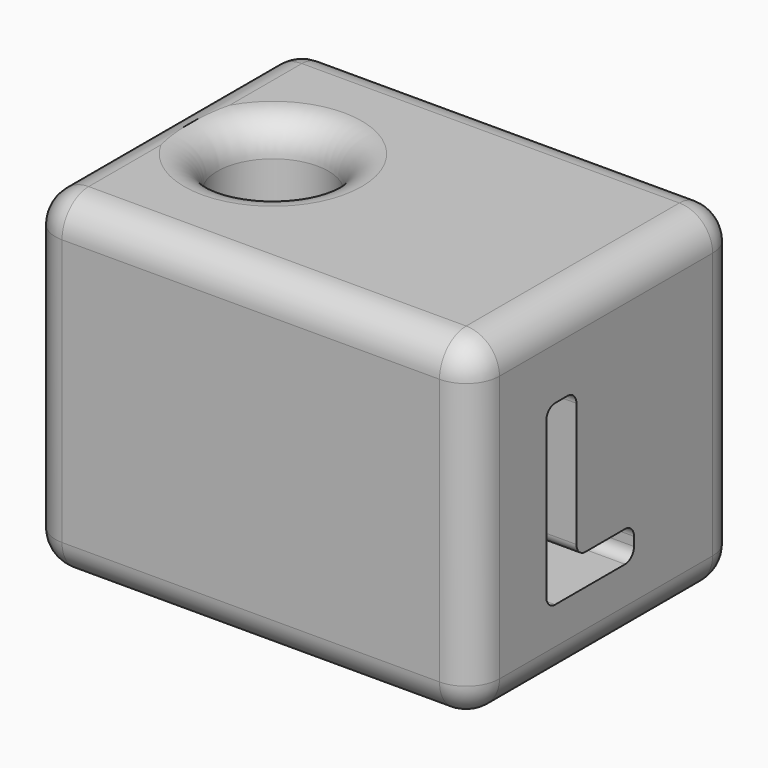
from build123d import *

# Parameters (mm, degrees)
F0_W         = 50.8
F0_H         = 38.1
F1_DEPTH     = 38.1
F2_R         = 6.35
F3_DEPTH     = 38.101
F4_T1_DEPTH  = 43.18
F4_T3_DEPTH  = 30.48
F4_T5_DEPTH  = 30.48
F4_S9_W      = 3.81
F4_S9_H      = 3.81
F4_T10_DEPTH = 3.81
F4_S15_W     = 3.81
F4_S15_H     = 3.81
F4_T16_DEPTH = 3.81
F4_S21_W     = 3.81
F4_S21_H     = 3.81
F4_T22_DEPTH = 3.81
F4_S27_W     = 3.81
F4_S27_H     = 3.81
F4_T28_DEPTH = 3.81
F4_S33_W     = 3.81
F4_S33_H     = 3.81
F4_T34_DEPTH = 3.81
F4_S39_W     = 3.81
F4_S39_H     = 3.81
F4_T40_DEPTH = 3.81
F4_S45_W     = 3.81
F4_S45_H     = 3.81
F4_T46_DEPTH = 3.81
F4_S51_W     = 3.81
F4_S51_H     = 3.81
F4_T52_DEPTH = 3.81
F5_TEXT_SIZE = 28.4437594625
F6_DEPTH     = 50.8010001
F7_R         = 1.27
F8_TEXT_SIZE = 26.0072152337
F9_DEPTH     = 1.27


# Not quite as in the source:
# - a fillet or chamfer that OpenCascade refuses, or shapes differently, is made with other operations: its cross-section is extruded or revolved along the edge and cut away or added
# - Text() gives the source's letters only with a copy of the font that has no kerning and outlines rounded to 1/6400 em; it was checked with that copy


with BuildPart() as f1:
    # F0 (on Top) → F1 (new body)
    with BuildSketch(Plane.XY):
        with Locations((25.4, 19.05)):
            Rectangle(F0_W, F0_H)
    extrude(amount=F1_DEPTH)

    # F2 (on face) → F3 (cut, through all)
    with BuildSketch(Plane.XY.offset(38.1)):
        with Locations((12.7, 19.05)):
            Circle(F2_R)
    extrude(amount=-F3_DEPTH, mode=Mode.SUBTRACT)

    # F4: fillet of radius 3.81 on 14 edges, made by hand

    # F4_s2 → F4_t1 (cut)
    with BuildSketch(Plane.YZ.offset(3.81)):
        with BuildLine():
            ThreePointArc((0, 34.29), (1.1159231637, 36.9840768363), (3.81, 38.1))
            Line((3.81, 38.1), (0, 38.1))
            Line((0, 38.1), (0, 34.29))
        make_face()
        with BuildLine():
            ThreePointArc((38.1, 34.29), (36.9840768363, 36.9840768363), (34.29, 38.1))
            Line((34.29, 38.1), (38.1, 38.1))
            Line((38.1, 38.1), (38.1, 34.29))
        make_face()
        with BuildLine():
            ThreePointArc((38.1, 3.81), (36.9840768363, 1.1159231637), (34.29, 0))
            Line((34.29, 0), (38.1, 0))
            Line((38.1, 0), (38.1, 3.81))
        make_face()
        with BuildLine():
            ThreePointArc((0, 3.81), (1.1159231637, 1.1159231637), (3.81, 0))
            Line((3.81, 0), (0, 0))
            Line((0, 0), (0, 3.81))
        make_face()
    extrude(amount=F4_T1_DEPTH, mode=Mode.SUBTRACT)

    # F4_s4 → F4_t3 (cut)
    with BuildSketch(Plane.XZ.offset(-34.29)):
        with BuildLine():
            ThreePointArc((0, 34.29), (1.1159231637, 36.9840768363), (3.81, 38.1))
            Line((3.81, 38.1), (0, 38.1))
            Line((0, 38.1), (0, 34.29))
        make_face()
        with BuildLine():
            ThreePointArc((46.99, 38.1), (49.6840768363, 36.9840768363), (50.8, 34.29))
            Line((50.8, 34.29), (50.8, 38.1))
            Line((50.8, 38.1), (46.99, 38.1))
        make_face()
        with BuildLine():
            ThreePointArc((0, 3.81), (1.1159231637, 1.1159231637), (3.81, 0))
            Line((3.81, 0), (0, 0))
            Line((0, 0), (0, 3.81))
        make_face()
        with BuildLine():
            ThreePointArc((46.99, 0), (49.6840768363, 1.1159231637), (50.8, 3.81))
            Line((50.8, 3.81), (50.8, 0))
            Line((50.8, 0), (46.99, 0))
        make_face()
    extrude(amount=F4_T3_DEPTH, mode=Mode.SUBTRACT)

    # F4_s6 → F4_t5 (cut)
    with BuildSketch(Plane.XY.offset(3.81)):
        with BuildLine():
            ThreePointArc((46.99, 0), (49.6840768363, 1.1159231637), (50.8, 3.81))
            Line((50.8, 3.81), (50.8, 0))
            Line((50.8, 0), (46.99, 0))
        make_face()
        with BuildLine():
            ThreePointArc((46.99, 38.1), (49.6840768363, 36.9840768363), (50.8, 34.29))
            Line((50.8, 34.29), (50.8, 38.1))
            Line((50.8, 38.1), (46.99, 38.1))
        make_face()
        with BuildLine():
            ThreePointArc((0, 34.29), (1.1159231637, 36.9840768363), (3.81, 38.1))
            Line((3.81, 38.1), (0, 38.1))
            Line((0, 38.1), (0, 34.29))
        make_face()
        with BuildLine():
            ThreePointArc((0, 3.81), (1.1159231637, 1.1159231637), (3.81, 0))
            Line((3.81, 0), (0, 0))
            Line((0, 0), (0, 3.81))
        make_face()
    extrude(amount=F4_T5_DEPTH, mode=Mode.SUBTRACT)


with BuildPart() as f4_tool8:
    # F4_s9 → F4_t10 (new body)
    with BuildSketch(Plane.YZ.offset(3.81)):
        with Locations((1.905, 36.195)):
            Rectangle(F4_S9_W, F4_S9_H)
    extrude(amount=-F4_T10_DEPTH)

    # F4_s11 → F4_t12 (revolve, cut)
    with BuildSketch(Plane(origin=(3.81, 3.81, 34.29), x_dir=(0, 0.7071067812, -0.7071067812), z_dir=(0, 0.7071067812, 0.7071067812))):
        with BuildLine():
            ThreePointArc((0, -3.81), (3.81, 0), (0, 3.81))
            Line((0, 3.81), (0, -3.81))
        make_face()
    revolve(axis=Axis((3.81, 3.81, 34.29), (-1, 0, 0)), mode=Mode.SUBTRACT)


with BuildPart() as f1_1:
    add(f1.part)

    # F4_t7: cut F4_tool8
    add(f4_tool8.part, mode=Mode.SUBTRACT)


with BuildPart() as f4_tool14:
    # F4_s15 → F4_t16 (new body)
    with BuildSketch(Plane.XZ.offset(-3.81)):
        with Locations((48.895, 36.195)):
            Rectangle(F4_S15_W, F4_S15_H)
    extrude(amount=F4_T16_DEPTH)

    # F4_s17 → F4_t18 (revolve, cut)
    with BuildSketch(Plane(origin=(46.99, 3.81, 34.29), x_dir=(-0.7071067812, 0, -0.7071067812), z_dir=(-0.7071067812, 0, 0.7071067812))):
        with BuildLine():
            ThreePointArc((0, -3.81), (3.81, 0), (0, 3.81))
            Line((0, 3.81), (0, -3.81))
        make_face()
    revolve(axis=Axis((46.99, 3.81, 34.29), (0, -1, 0)), mode=Mode.SUBTRACT)


with BuildPart() as f1_2:
    add(f1_1.part)

    # F4_t13: cut F4_tool14
    add(f4_tool14.part, mode=Mode.SUBTRACT)


with BuildPart() as f4_tool20:
    # F4_s21 → F4_t22 (new body)
    with BuildSketch(Plane.YZ.offset(3.81)):
        with Locations((36.195, 36.195)):
            Rectangle(F4_S21_W, F4_S21_H)
    extrude(amount=-F4_T22_DEPTH)

    # F4_s23 → F4_t24 (revolve, cut)
    with BuildSketch(Plane(origin=(3.81, 34.29, 34.29), x_dir=(0, -0.7071067812, -0.7071067812), z_dir=(0, 0.7071067812, -0.7071067812))):
        with BuildLine():
            ThreePointArc((0, -3.81), (3.81, 0), (0, 3.81))
            Line((0, 3.81), (0, -3.81))
        make_face()
    revolve(axis=Axis((3.81, 34.29, 34.29), (-1, 0, 0)), mode=Mode.SUBTRACT)


with BuildPart() as f1_3:
    add(f1_2.part)

    # F4_t19: cut F4_tool20
    add(f4_tool20.part, mode=Mode.SUBTRACT)


with BuildPart() as f4_tool26:
    # F4_s27 → F4_t28 (new body)
    with BuildSketch(Plane.XZ.offset(-34.29)):
        with Locations((48.895, 36.195)):
            Rectangle(F4_S27_W, F4_S27_H)
    extrude(amount=-F4_T28_DEPTH)

    # F4_s29 → F4_t30 (revolve, cut)
    with BuildSketch(Plane(origin=(46.99, 34.29, 34.29), x_dir=(-0.7071067812, 0, -0.7071067812), z_dir=(0.7071067812, 0, -0.7071067812))):
        with BuildLine():
            ThreePointArc((0, -3.81), (3.81, 0), (0, 3.81))
            Line((0, 3.81), (0, -3.81))
        make_face()
    revolve(axis=Axis((46.99, 34.29, 34.29), (0, 1, 0)), mode=Mode.SUBTRACT)


with BuildPart() as f1_4:
    add(f1_3.part)

    # F4_t25: cut F4_tool26
    add(f4_tool26.part, mode=Mode.SUBTRACT)


with BuildPart() as f4_tool32:
    # F4_s33 → F4_t34 (new body)
    with BuildSketch(Plane.XZ.offset(-34.29)):
        with Locations((48.895, 1.905)):
            Rectangle(F4_S33_W, F4_S33_H)
    extrude(amount=-F4_T34_DEPTH)

    # F4_s35 → F4_t36 (revolve, cut)
    with BuildSketch(Plane(origin=(46.99, 34.29, 3.81), x_dir=(-0.7071067812, 0, 0.7071067812), z_dir=(-0.7071067812, 0, -0.7071067812))):
        with BuildLine():
            ThreePointArc((0, -3.81), (3.81, 0), (0, 3.81))
            Line((0, 3.81), (0, -3.81))
        make_face()
    revolve(axis=Axis((46.99, 34.29, 3.81), (0, 1, 0)), mode=Mode.SUBTRACT)


with BuildPart() as f1_5:
    add(f1_4.part)

    # F4_t31: cut F4_tool32
    add(f4_tool32.part, mode=Mode.SUBTRACT)


with BuildPart() as f4_tool38:
    # F4_s39 → F4_t40 (new body)
    with BuildSketch(Plane.YZ.offset(3.81)):
        with Locations((36.195, 1.905)):
            Rectangle(F4_S39_W, F4_S39_H)
    extrude(amount=-F4_T40_DEPTH)

    # F4_s41 → F4_t42 (revolve, cut)
    with BuildSketch(Plane(origin=(3.81, 34.29, 3.81), x_dir=(0, -0.7071067812, 0.7071067812), z_dir=(0, -0.7071067812, -0.7071067812))):
        with BuildLine():
            ThreePointArc((0, -3.81), (3.81, 0), (0, 3.81))
            Line((0, 3.81), (0, -3.81))
        make_face()
    revolve(axis=Axis((3.81, 34.29, 3.81), (-1, 0, 0)), mode=Mode.SUBTRACT)


with BuildPart() as f1_6:
    add(f1_5.part)

    # F4_t37: cut F4_tool38
    add(f4_tool38.part, mode=Mode.SUBTRACT)


with BuildPart() as f4_tool44:
    # F4_s45 → F4_t46 (new body)
    with BuildSketch(Plane.YZ.offset(3.81)):
        with Locations((1.905, 1.905)):
            Rectangle(F4_S45_W, F4_S45_H)
    extrude(amount=-F4_T46_DEPTH)

    # F4_s47 → F4_t48 (revolve, cut)
    with BuildSketch(Plane(origin=(3.81, 3.81, 3.81), x_dir=(0, 0.7071067812, 0.7071067812), z_dir=(0, -0.7071067812, 0.7071067812))):
        with BuildLine():
            ThreePointArc((0, -3.81), (3.81, 0), (0, 3.81))
            Line((0, 3.81), (0, -3.81))
        make_face()
    revolve(axis=Axis((3.81, 3.81, 3.81), (-1, 0, 0)), mode=Mode.SUBTRACT)


with BuildPart() as f1_7:
    add(f1_6.part)

    # F4_t43: cut F4_tool44
    add(f4_tool44.part, mode=Mode.SUBTRACT)


with BuildPart() as f4_tool50:
    # F4_s51 → F4_t52 (new body)
    with BuildSketch(Plane.XZ.offset(-3.81)):
        with Locations((48.895, 1.905)):
            Rectangle(F4_S51_W, F4_S51_H)
    extrude(amount=F4_T52_DEPTH)

    # F4_s53 → F4_t54 (revolve, cut)
    with BuildSketch(Plane(origin=(46.99, 3.81, 3.81), x_dir=(-0.7071067812, 0, 0.7071067812), z_dir=(0.7071067812, 0, 0.7071067812))):
        with BuildLine():
            ThreePointArc((0, -3.81), (3.81, 0), (0, 3.81))
            Line((0, 3.81), (0, -3.81))
        make_face()
    revolve(axis=Axis((46.99, 3.81, 3.81), (0, -1, 0)), mode=Mode.SUBTRACT)


with BuildPart() as f1_8:
    add(f1_7.part)

    # F4_t49: cut F4_tool50
    add(f4_tool50.part, mode=Mode.SUBTRACT)

    # F4_s55 → F4_t56 (revolve, cut)
    with BuildSketch(Plane.XZ.offset(-19.05)):
        with BuildLine():
            ThreePointArc((22.86, 0), (20.1659231637, 1.1159231637), (19.05, 3.81))
            Line((19.05, 3.81), (19.05, 0))
            Line((19.05, 0), (22.86, 0))
        make_face()
    revolve(axis=Axis((12.7, 19.05, 0), (0, 0, 1)), mode=Mode.SUBTRACT)

    # F4_s57 → F4_t58 (revolve, cut)
    with BuildSketch(Plane.XZ.offset(-19.05)):
        with BuildLine():
            ThreePointArc((22.86, 38.1), (20.1659231637, 36.9840768363), (19.05, 34.29))
            Line((19.05, 34.29), (19.05, 38.1))
            Line((19.05, 38.1), (22.86, 38.1))
        make_face()
    revolve(axis=Axis((12.7, 19.05, 38.1), (0, 0, 1)), mode=Mode.SUBTRACT)

    # F5 (on face) → F6 (cut, through all)
    with BuildSketch(Plane.YZ.offset(50.8)):
        with Locations((7.9516330734, 8.0470358953)):
            Text('L', F5_TEXT_SIZE, font='Open Sans', font_style=FontStyle.BOLD, text_align=(TextAlign.LEFT, TextAlign.BOTTOM))
    extrude(amount=-F6_DEPTH, mode=Mode.SUBTRACT)

    # F7
    f7_edges = [f1_8.edges().sort_by_distance(p)[0] for p in [
        (25.4, 10.507127, 28.353214),
        (34.115173, 14.81369, 28.353214),
        (34.115173, 14.81369, 11.602506),
        (34.216279, 23.049047, 11.602506),
        (34.216279, 23.049047, 8.047036),
        (25.4, 10.507127, 8.047036),
        (3.984827, 14.81369, 28.353214),
        (3.984827, 14.81369, 11.602506),
        (3.883721, 23.049047, 11.602506),
        (3.883721, 23.049047, 8.047036),
    ]]
    fillet(f7_edges, radius=F7_R)

    # F8 (on face) → F9 (join)
    with BuildSketch(Plane(origin=(0, 38.1, 0), x_dir=(-1, 0, 0), z_dir=(0, 1, 0))):
        with Locations((-45.7914285362, 10.8914086595)):
            Text('evi', F8_TEXT_SIZE, font='Open Sans', text_align=(TextAlign.LEFT, TextAlign.BOTTOM))
    extrude(amount=F9_DEPTH)


solid = f1_8.part
